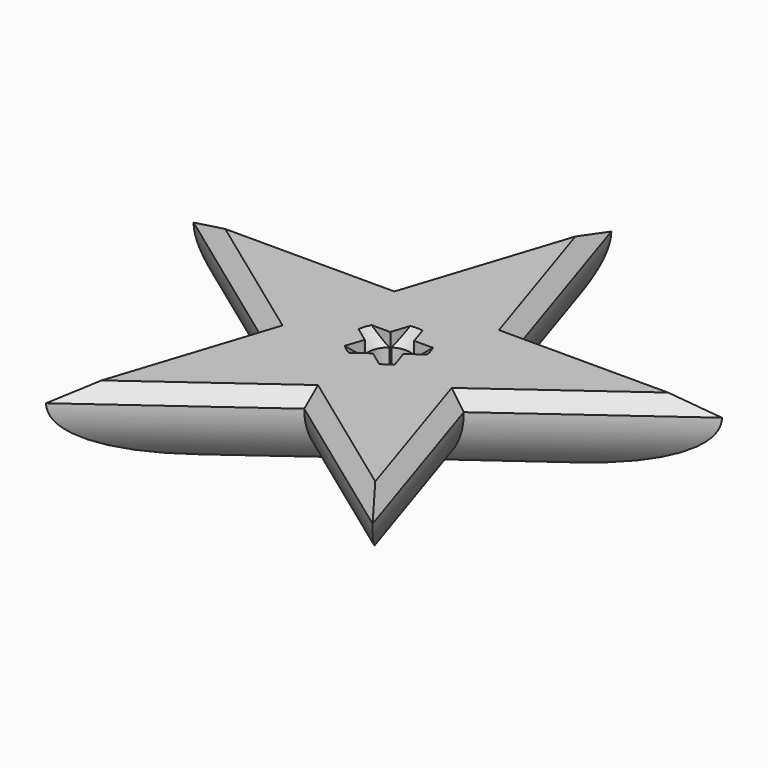
from build123d import *

# Parameters (mm, degrees)
F1_DEPTH     = 30
F2_SIZE      = 5
F3_R         = 24.99999
F5_DEPTH     = 35
F6_T4_ANGLE  = 264.2993733481
F6_T11_ANGLE = 264.2993733481
F6_T18_ANGLE = 264.2993733481
F6_T24_ANGLE = 264.2993733481
F6_T30_ANGLE = 264.2993733481
F6_T37_ANGLE = 264.2993733481
F6_T44_ANGLE = 264.2993733481
F6_T51_ANGLE = 264.2993733481
F6_T57_ANGLE = 264.2993733481
F6_T63_ANGLE = 264.2993733481
F6_T70_ANGLE = 264.299373348
F6_T77_ANGLE = 264.299373348
F6_T84_ANGLE = 264.299373348


# Not quite as in the source:
# - a fillet or chamfer that OpenCascade refuses, or shapes differently, is made with other operations: its cross-section is extruded or revolved along the edge and cut away or added
# - a fillet or chamfer is up to 0.001 mm smaller than in the source, because OpenCascade refuses the exact size


with BuildPart() as f1:
    # F0 (on Top) → F1 (new body)
    with BuildSketch(Plane.XY):
        Polygon((22.451398829, 30.9016994375), (0, 100), (-22.451398829, 30.9016994375), (-95.1056516295, 30.9016994375), (-36.3271264003, -11.803398875), (-58.7785252292, -80.9016994375), (0, -38.196601125), (58.7785252292, -80.9016994375), (36.3271264003, -11.803398875), (95.1056516295, 30.9016994375), align=None)
    extrude(amount=F1_DEPTH)

    # F2
    f2_edges = [f1.edges().sort_by_distance(p)[0] for p in [
        (65.716389, 9.54915, 30),
        (58.778525, 30.901699, 30),
        (11.225699, 65.45085, 30),
        (-11.225699, 65.45085, 30),
        (-58.778525, 30.901699, 30),
        (-65.716389, 9.54915, 30),
        (-47.552826, -46.352549, 30),
        (-29.389263, -59.54915, 30),
        (29.389263, -59.54915, 30),
        (47.552826, -46.352549, 30),
    ]]
    chamfer(f2_edges, length=F2_SIZE)

    # F3 (radius 25 in the source; OpenCascade refuses exactly that, so slightly less here)
    f3_edges = [f1.edges().sort_by_distance(p)[0] for p in [
        (65.716389, 9.54915, 0),
        (58.778525, 30.901699, 0),
        (11.225699, 65.45085, 0),
        (-11.225699, 65.45085, 0),
        (-58.778525, 30.901699, 0),
        (-65.716389, 9.54915, 0),
        (-47.552826, -46.352549, 0),
        (-29.389263, -59.54915, 0),
        (29.389263, -59.54915, 0),
        (47.552826, -46.352549, 0),
    ]]
    fillet(f3_edges, radius=F3_R)

    # F4 (on face) → F5 (cut)
    with BuildSketch(Plane(origin=(0, 0, 0), x_dir=(1, 0, 0), z_dir=(0, 0, -1))):
        with BuildLine():
            ThreePointArc((4.6281557575, -5.9017094375), (6.7439294251, -3.2816788249), (7.5, 0))
            ThreePointArc((7.5, 0), (7.4279525521, 1.0370732295), (7.2131944311, 2.0542215312))
            Line((7.2131944311, 2.0542215312), (6.9378755413, 2.2542524134))
            Line((6.9378755413, 2.2542524134), (7.0430379995, 2.5779091795))
            ThreePointArc((7.0430379995, 2.5779091795), (4.4083893922, 6.0676274578), (0.2753188897, 7.4949449303))
            Line((0.2753188897, 7.4949449303), (0, 7.2949140482))
            Line((0, 7.2949140482), (-0.2753188897, 7.4949449303))
            ThreePointArc((-0.2753188897, 7.4949449303), (-4.4083893922, 6.0676274578), (-7.0430379995, 2.5779091795))
            Line((-7.0430379995, 2.5779091795), (-6.9378755413, 2.2542524134))
            Line((-6.9378755413, 2.2542524134), (-7.2131944311, 2.0542215312))
            ThreePointArc((-7.2131944311, 2.0542215312), (-7.1329238722, -2.3176274578), (-4.6281557575, -5.9017094375))
            Line((-4.6281557575, -5.9017094375), (-4.2878428943, -5.9017094375))
            Line((-4.2878428943, -5.9017094375), (-4.1826804361, -6.2253662036))
            ThreePointArc((-4.1826804361, -6.2253662036), (0, -7.5), (4.1826804361, -6.2253662036))
            Line((4.1826804361, -6.2253662036), (4.2878428943, -5.9017094375))
            Line((4.2878428943, -5.9017094375), (4.6281557575, -5.9017094375))
        make_face()
    extrude(amount=-F5_DEPTH, mode=Mode.SUBTRACT)

    # F6: chamfer of 5 on 5 edges, made by hand


with BuildPart() as f6_tool2:
    # F6_s3 → F6_t4 (revolve)
    with BuildSketch(Plane(origin=(0, 0, 0), x_dir=(0, 0, 1), z_dir=(0.9124797315, 0.4091219129, 0))):
        Polygon((30, 12.5), (25, 7.5), (30, 7.5), align=None)
    revolve(axis=Axis((0, 0, 30), (0, 0, -1)), revolution_arc=F6_T4_ANGLE)

    split(bisect_by=Plane(origin=(-5.6128592178, 1.823728512, 0), x_dir=(0, 0, 1), z_dir=(0.9510565163, -0.3090169944, 0)), keep=Keep.TOP)

    split(bisect_by=Plane(origin=(-3.4689377707, -4.7745832308, 0), x_dir=(0, 0, 1), z_dir=(0.5877852523, 0.8090169944, 0)), keep=Keep.TOP)

    split(bisect_by=Plane(origin=(5.6128592178, 1.823728512, 0), x_dir=(0, 0, 1), z_dir=(-0.9510565163, -0.3090169944, 0)), keep=Keep.TOP)


with BuildPart() as f1_1:
    add(f1.part)

    # F6_t1: cut F6_tool2
    add(f6_tool2.part, mode=Mode.SUBTRACT)


with BuildPart() as f6_tool9:
    # F6_s10 → F6_t11 (revolve)
    with BuildSketch(Plane(origin=(0, 0, 0), x_dir=(0, 0, 1), z_dir=(0.9124797315, 0.4091219129, 0))):
        Polygon((30, 12.5), (25, 7.5), (30, 7.5), align=None)
    revolve(axis=Axis((0, 0, 30), (0, 0, -1)), revolution_arc=F6_T11_ANGLE)

    split(bisect_by=Plane.XZ.offset(-5.9017094375), keep=Keep.TOP)

    split(bisect_by=Plane(origin=(-5.6128592178, 1.823728512, 0), x_dir=(0, 0, 1), z_dir=(0.9510565163, -0.3090169944, 0)), keep=Keep.TOP)

    split(bisect_by=Plane(origin=(3.4689377707, -4.7745832308, 0), x_dir=(0, 0, 1), z_dir=(-0.5877852523, 0.8090169944, 0)), keep=Keep.TOP)


with BuildPart() as f1_2:
    add(f1_1.part)

    # F6_t8: cut F6_tool9
    add(f6_tool9.part, mode=Mode.SUBTRACT)


with BuildPart() as f6_tool16:
    # F6_s17 → F6_t18 (revolve)
    with BuildSketch(Plane(origin=(0, 0, 0), x_dir=(0, 0, 1), z_dir=(0.9124797315, 0.4091219129, 0))):
        Polygon((30, 12.5), (25, 7.5), (30, 7.5), align=None)
    revolve(axis=Axis((0, 0, 30), (0, 0, -1)), revolution_arc=F6_T18_ANGLE)

    split(bisect_by=Plane.XZ.offset(-5.9017094375), keep=Keep.TOP)

    split(bisect_by=Plane(origin=(-3.4689377707, -4.7745832308, 0), x_dir=(0, 0, 1), z_dir=(0.5877852523, 0.8090169944, 0)), keep=Keep.TOP)


with BuildPart() as f1_3:
    add(f1_2.part)

    # F6_t15: cut F6_tool16
    add(f6_tool16.part, mode=Mode.SUBTRACT)


with BuildPart() as f6_tool22:
    # F6_s23 → F6_t24 (revolve)
    with BuildSketch(Plane(origin=(0, 0, 0), x_dir=(0, 0, 1), z_dir=(0.6710698053, -0.7413941707, 0))):
        Polygon((30, 12.5), (25, 7.5), (30, 7.5), align=None)
    revolve(axis=Axis((0, 0, 30), (0, 0, -1)), revolution_arc=F6_T24_ANGLE)

    split(bisect_by=Plane(origin=(5.6128592178, 1.823728512, 0), x_dir=(0, 0, 1), z_dir=(-0.9510565163, -0.3090169944, 0)), keep=Keep.TOP)

    split(bisect_by=Plane(origin=(-5.6128592178, 1.823728512, 0), x_dir=(0, 0, 1), z_dir=(0.9510565163, -0.3090169944, 0)), keep=Keep.TOP)


with BuildPart() as f1_4:
    add(f1_3.part)

    # F6_t21: cut F6_tool22
    add(f6_tool22.part, mode=Mode.SUBTRACT)


with BuildPart() as f6_tool28:
    # F6_s29 → F6_t30 (revolve)
    with BuildSketch(Plane(origin=(0, 0, 0), x_dir=(0, 0, 1), z_dir=(0.6710698053, -0.7413941707, 0))):
        Polygon((30, 12.5), (25, 7.5), (30, 7.5), align=None)
    revolve(axis=Axis((0, 0, 30), (0, 0, -1)), revolution_arc=F6_T30_ANGLE)

    split(bisect_by=Plane(origin=(3.4689377707, -4.7745832308, 0), x_dir=(0, 0, 1), z_dir=(-0.5877852523, 0.8090169944, 0)), keep=Keep.TOP)

    split(bisect_by=Plane.XZ.offset(-5.9017094375), keep=Keep.TOP)

    split(bisect_by=Plane(origin=(-3.4689377707, -4.7745832308, 0), x_dir=(0, 0, 1), z_dir=(0.5877852523, 0.8090169944, 0)), keep=Keep.TOP)


with BuildPart() as f1_5:
    add(f1_4.part)

    # F6_t27: cut F6_tool28
    add(f6_tool28.part, mode=Mode.SUBTRACT)


with BuildPart() as f6_tool35:
    # F6_s36 → F6_t37 (revolve)
    with BuildSketch(Plane(origin=(0, 0, 0), x_dir=(0, 0, 1), z_dir=(-0.497735783, -0.8673287095, 0))):
        Polygon((30, 12.5), (25, 7.5), (30, 7.5), align=None)
    revolve(axis=Axis((0, 0, 30), (0, 0, -1)), revolution_arc=F6_T37_ANGLE)

    split(bisect_by=Plane(origin=(5.6128592178, 1.823728512, 0), x_dir=(0, 0, 1), z_dir=(-0.9510565163, -0.3090169944, 0)), keep=Keep.TOP)

    split(bisect_by=Plane.XZ.offset(-5.9017094375), keep=Keep.TOP)

    split(bisect_by=Plane(origin=(-3.4689377707, -4.7745832308, 0), x_dir=(0, 0, 1), z_dir=(0.5877852523, 0.8090169944, 0)), keep=Keep.TOP)


with BuildPart() as f1_6:
    add(f1_5.part)

    # F6_t34: cut F6_tool35
    add(f6_tool35.part, mode=Mode.SUBTRACT)


with BuildPart() as f6_tool42:
    # F6_s43 → F6_t44 (revolve)
    with BuildSketch(Plane(origin=(0, 0, 0), x_dir=(0, 0, 1), z_dir=(-0.497735783, -0.8673287095, 0))):
        Polygon((30, 12.5), (25, 7.5), (30, 7.5), align=None)
    revolve(axis=Axis((0, 0, 30), (0, 0, -1)), revolution_arc=F6_T44_ANGLE)

    split(bisect_by=Plane(origin=(3.4689377707, -4.7745832308, 0), x_dir=(0, 0, 1), z_dir=(-0.5877852523, 0.8090169944, 0)), keep=Keep.TOP)

    split(bisect_by=Plane(origin=(5.6128592178, 1.823728512, 0), x_dir=(0, 0, 1), z_dir=(-0.9510565163, -0.3090169944, 0)), keep=Keep.TOP)

    split(bisect_by=Plane(origin=(-5.6128592178, 1.823728512, 0), x_dir=(0, 0, 1), z_dir=(0.9510565163, -0.3090169944, 0)), keep=Keep.TOP)


with BuildPart() as f1_7:
    add(f1_6.part)

    # F6_t41: cut F6_tool42
    add(f6_tool42.part, mode=Mode.SUBTRACT)


with BuildPart() as f6_tool49:
    # F6_s50 → F6_t51 (revolve)
    with BuildSketch(Plane(origin=(0, 0, 0), x_dir=(0, 0, 1), z_dir=(-0.497735783, -0.8673287095, 0))):
        Polygon((30, 12.5), (25, 7.5), (30, 7.5), align=None)
    revolve(axis=Axis((0, 0, 30), (0, 0, -1)), revolution_arc=F6_T51_ANGLE)

    split(bisect_by=Plane(origin=(3.4689377707, -4.7745832308, 0), x_dir=(0, 0, 1), z_dir=(-0.5877852523, 0.8090169944, 0)), keep=Keep.TOP)

    split(bisect_by=Plane.XZ.offset(-5.9017094375), keep=Keep.TOP)


with BuildPart() as f1_8:
    add(f1_7.part)

    # F6_t48: cut F6_tool49
    add(f6_tool49.part, mode=Mode.SUBTRACT)


with BuildPart() as f6_tool55:
    # F6_s56 → F6_t57 (revolve)
    with BuildSketch(Plane(origin=(0, 0, 0), x_dir=(0, 0, 1), z_dir=(-0.9786874366, 0.2053555488, 0))):
        Polygon((30, 12.5), (25, 7.5), (30, 7.5), align=None)
    revolve(axis=Axis((0, 0, 30), (0, 0, -1)), revolution_arc=F6_T57_ANGLE)

    split(bisect_by=Plane(origin=(5.6128592178, 1.823728512, 0), x_dir=(0, 0, 1), z_dir=(-0.9510565163, -0.3090169944, 0)), keep=Keep.TOP)

    split(bisect_by=Plane(origin=(-3.4689377707, -4.7745832308, 0), x_dir=(0, 0, 1), z_dir=(0.5877852523, 0.8090169944, 0)), keep=Keep.TOP)


with BuildPart() as f1_9:
    add(f1_8.part)

    # F6_t54: cut F6_tool55
    add(f6_tool55.part, mode=Mode.SUBTRACT)


with BuildPart() as f6_tool61:
    # F6_s62 → F6_t63 (revolve)
    with BuildSketch(Plane(origin=(0, 0, 0), x_dir=(0, 0, 1), z_dir=(-0.9786874366, 0.2053555488, 0))):
        Polygon((30, 12.5), (25, 7.5), (30, 7.5), align=None)
    revolve(axis=Axis((0, 0, 30), (0, 0, -1)), revolution_arc=F6_T63_ANGLE)

    split(bisect_by=Plane(origin=(3.4689377707, -4.7745832308, 0), x_dir=(0, 0, 1), z_dir=(-0.5877852523, 0.8090169944, 0)), keep=Keep.TOP)

    split(bisect_by=Plane.XZ.offset(-5.9017094375), keep=Keep.TOP)

    split(bisect_by=Plane(origin=(-5.6128592178, 1.823728512, 0), x_dir=(0, 0, 1), z_dir=(0.9510565163, -0.3090169944, 0)), keep=Keep.TOP)


with BuildPart() as f1_10:
    add(f1_9.part)

    # F6_t60: cut F6_tool61
    add(f6_tool61.part, mode=Mode.SUBTRACT)


with BuildPart() as f6_tool68:
    # F6_s69 → F6_t70 (revolve)
    with BuildSketch(Plane(origin=(0, 0, 0), x_dir=(0, 0, 1), z_dir=(-0.1071263172, 0.9942454185, 0))):
        Polygon((30, 12.5), (25, 7.5), (30, 7.5), align=None)
    revolve(axis=Axis((0, 0, 30), (0, 0, -1)), revolution_arc=F6_T70_ANGLE)

    split(bisect_by=Plane(origin=(3.4689377707, -4.7745832308, 0), x_dir=(0, 0, 1), z_dir=(-0.5877852523, 0.8090169944, 0)), keep=Keep.TOP)

    split(bisect_by=Plane(origin=(-3.4689377707, -4.7745832308, 0), x_dir=(0, 0, 1), z_dir=(0.5877852523, 0.8090169944, 0)), keep=Keep.TOP)

    split(bisect_by=Plane.XZ.offset(-5.9017094375), keep=Keep.TOP)


with BuildPart() as f1_11:
    add(f1_10.part)

    # F6_t67: cut F6_tool68
    add(f6_tool68.part, mode=Mode.SUBTRACT)


with BuildPart() as f6_tool75:
    # F6_s76 → F6_t77 (revolve)
    with BuildSketch(Plane(origin=(0, 0, 0), x_dir=(0, 0, 1), z_dir=(-0.1071263172, 0.9942454185, 0))):
        Polygon((30, 12.5), (25, 7.5), (30, 7.5), align=None)
    revolve(axis=Axis((0, 0, 30), (0, 0, -1)), revolution_arc=F6_T77_ANGLE)

    split(bisect_by=Plane(origin=(5.6128592178, 1.823728512, 0), x_dir=(0, 0, 1), z_dir=(-0.9510565163, -0.3090169944, 0)), keep=Keep.TOP)

    split(bisect_by=Plane(origin=(-5.6128592178, 1.823728512, 0), x_dir=(0, 0, 1), z_dir=(0.9510565163, -0.3090169944, 0)), keep=Keep.TOP)

    split(bisect_by=Plane(origin=(-3.4689377707, -4.7745832308, 0), x_dir=(0, 0, 1), z_dir=(0.5877852523, 0.8090169944, 0)), keep=Keep.TOP)


with BuildPart() as f1_12:
    add(f1_11.part)

    # F6_t74: cut F6_tool75
    add(f6_tool75.part, mode=Mode.SUBTRACT)


with BuildPart() as f6_tool82:
    # F6_s83 → F6_t84 (revolve)
    with BuildSketch(Plane(origin=(0, 0, 0), x_dir=(0, 0, 1), z_dir=(-0.1071263172, 0.9942454185, 0))):
        Polygon((30, 12.5), (25, 7.5), (30, 7.5), align=None)
    revolve(axis=Axis((0, 0, 30), (0, 0, -1)), revolution_arc=F6_T84_ANGLE)

    split(bisect_by=Plane(origin=(3.4689377707, -4.7745832308, 0), x_dir=(0, 0, 1), z_dir=(-0.5877852523, 0.8090169944, 0)), keep=Keep.TOP)

    split(bisect_by=Plane(origin=(-5.6128592178, 1.823728512, 0), x_dir=(0, 0, 1), z_dir=(0.9510565163, -0.3090169944, 0)), keep=Keep.TOP)


with BuildPart() as f1_13:
    add(f1_12.part)

    # F6_t81: cut F6_tool82
    add(f6_tool82.part, mode=Mode.SUBTRACT)


solid = f1_13.part
